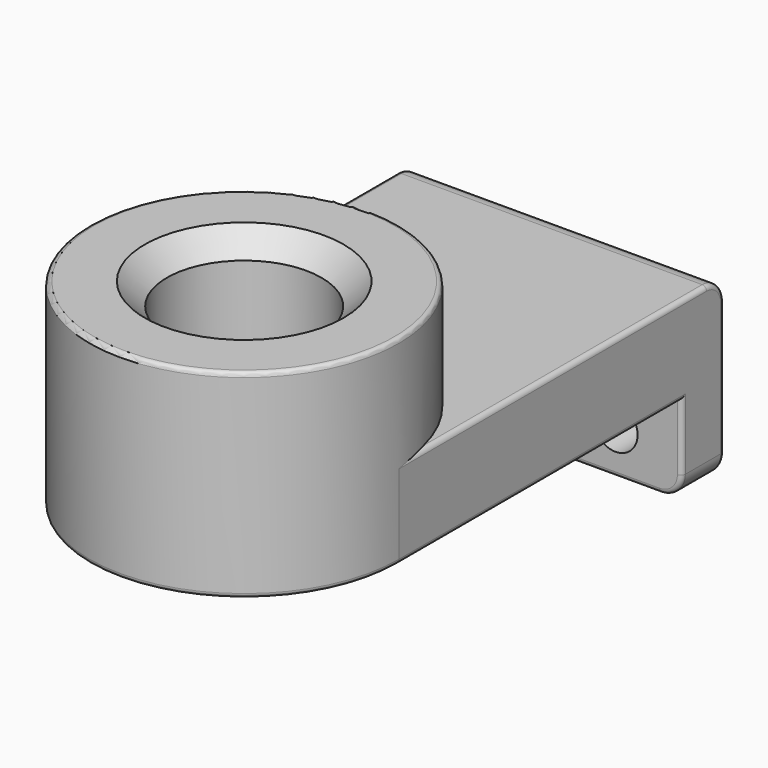
from build123d import *

# Parameters (mm, degrees)
F1_DEPTH     = 45
F2_DEPTH     = 20
F3_W         = 70
F3_H         = 20
F3_R         = 5
F4_DEPTH     = 12
F5_SIZE      = 5
F6_SIZE      = 5
F7_R         = 5
F8_T1_DEPTH  = 80
F8_T3_DEPTH  = 60
F8_T5_DEPTH  = 30
F8_T7_DEPTH  = 15
F8_T12_DEPTH = 99.5
F8_S13_R     = 35
F8_T14_DEPTH = 51
F8_T16_ANGLE = 180
F8_T20_DEPTH = 99.5
F8_S21_R     = 35
F8_T22_DEPTH = 51
F8_T24_ANGLE = 90
F8_T26_ANGLE = 90
F8_T28_ANGLE = 90
F8_T30_ANGLE = 90
F8_T32_ANGLE = 90
F8_T34_ANGLE = 90
F8_T39_DEPTH = 82.5
F8_T43_DEPTH = 17.5
F8_T50_DEPTH = 82.5
F8_T54_DEPTH = 17.5
F9_R         = 1


# Not quite as in the source:
# - a fillet or chamfer that OpenCascade refuses, or shapes differently, is made with other operations: its cross-section is extruded or revolved along the edge and cut away or added


with BuildPart() as f1:
    # F0 (on Top) → F1 (new body)
    with BuildSketch(Plane.XY):
        with BuildLine():
            Line((-23.7085466087, -49.8320348561), (-6.2085466087, -49.8320348561))
            ThreePointArc((-6.2085466087, -49.8320348561), (-41.2085466087, -14.8320348561), (-76.2085466087, -49.8320348561))
            Line((-76.2085466087, -49.8320348561), (-58.7085466087, -49.8320348561))
            ThreePointArc((-58.7085466087, -49.8320348561), (-41.2085466087, -32.3320348561), (-23.7085466087, -49.8320348561))
        make_face()
        with BuildLine():
            ThreePointArc((-76.2085466087, -49.8320348561), (-41.2085466087, -84.8320348561), (-6.2085466087, -49.8320348561))
            Line((-6.2085466087, -49.8320348561), (-23.7085466087, -49.8320348561))
            ThreePointArc((-23.7085466087, -49.8320348561), (-41.2085466087, -67.3320348561), (-58.7085466087, -49.8320348561))
            Line((-58.7085466087, -49.8320348561), (-76.2085466087, -49.8320348561))
        make_face()
    extrude(amount=F1_DEPTH)

    # F0 (on Top) → F2 (join)
    with BuildSketch(Plane.XY):
        with BuildLine():
            Line((-23.7085466087, -49.8320348561), (-6.2085466087, -49.8320348561))
            ThreePointArc((-6.2085466087, -49.8320348561), (-41.2085466087, -14.8320348561), (-76.2085466087, -49.8320348561))
            Line((-76.2085466087, -49.8320348561), (-58.7085466087, -49.8320348561))
            ThreePointArc((-58.7085466087, -49.8320348561), (-41.2085466087, -32.3320348561), (-23.7085466087, -49.8320348561))
        make_face()
        with BuildLine():
            ThreePointArc((-76.2085466087, -49.8320348561), (-41.2085466087, -84.8320348561), (-6.2085466087, -49.8320348561))
            Line((-6.2085466087, -49.8320348561), (-23.7085466087, -49.8320348561))
            ThreePointArc((-23.7085466087, -49.8320348561), (-41.2085466087, -67.3320348561), (-58.7085466087, -49.8320348561))
            Line((-58.7085466087, -49.8320348561), (-76.2085466087, -49.8320348561))
        make_face()
        with BuildLine():
            ThreePointArc((-76.2085466087, -49.8320348561), (-41.2085466087, -14.8320348561), (-6.2085466087, -49.8320348561))
            Line((-6.2085466087, -49.8320348561), (-6.2085466087, 30.1679651439))
            Line((-6.2085466087, 30.1679651439), (-76.2085466087, 30.1679651439))
            Line((-76.2085466087, 30.1679651439), (-76.2085466087, -49.8320348561))
        make_face()
    extrude(amount=F2_DEPTH)

    # F3 (on face) → F4 (join)
    with BuildSketch(Plane(origin=(0, 30.1679651439, 0), x_dir=(-1, 0, 0), z_dir=(0, 1, 0))):
        with Locations((41.2085466087, -10)):
            Rectangle(F3_W, F3_H)
        with BuildLine():
            ThreePointArc((21.2085466087, -5), (24.7440805146, -6.4644660941), (26.2085466087, -10))
            ThreePointArc((26.2085466087, -10), (17.6730127028, -13.5355339059), (21.2085466087, -5))
        make_face(mode=Mode.SUBTRACT)
        with Locations((61.2085466087, -10)):
            Circle(F3_R, mode=Mode.SUBTRACT)
        with Locations((41.2085466087, 10)):
            Rectangle(F3_W, F3_H)
    extrude(amount=F4_DEPTH)

    # F5
    f5_edges = [f1.edges().sort_by_distance(p)[0] for p in [
        (-58.708547, -49.832035, 45),
    ]]
    chamfer(f5_edges, length=F5_SIZE)

    # F6
    f6_edges = [f1.edges().sort_by_distance(p)[0] for p in [
        (-58.708547, -49.832035, 0),
    ]]
    chamfer(f6_edges, length=F6_SIZE)

    # F7
    f7_edges = [f1.edges().sort_by_distance(p)[0] for p in [
        (-76.208547, 36.167965, -20),
        (-6.208547, 36.167965, -20),
        (-41.208547, 42.167965, 20),
    ]]
    fillet(f7_edges, radius=F7_R)

    # F8: fillet of radius 1 on 9 edges, made by hand

    # F8_s2 → F8_t1 (cut)
    with BuildSketch(Plane.XZ.offset(-30.1679651439)):
        with BuildLine():
            ThreePointArc((-75.2085466087, 0), (-75.9156533899, 0.2928932188), (-76.2085466087, 1))
            Line((-76.2085466087, 1), (-76.2085466087, 0))
            Line((-76.2085466087, 0), (-75.2085466087, 0))
        make_face()
        with BuildLine():
            ThreePointArc((-6.2085466087, 1), (-6.5014398275, 0.2928932188), (-7.2085466087, 0))
            Line((-7.2085466087, 0), (-6.2085466087, 0))
            Line((-6.2085466087, 0), (-6.2085466087, 1))
        make_face()
    extrude(amount=F8_T1_DEPTH, mode=Mode.SUBTRACT)

    # F8_s4 → F8_t3 (cut)
    with BuildSketch(Plane.YZ.offset(-71.2085466087)):
        with BuildLine():
            ThreePointArc((30.1679651439, -19), (30.4608583627, -19.7071067812), (31.1679651439, -20))
            Line((31.1679651439, -20), (30.1679651439, -20))
            Line((30.1679651439, -20), (30.1679651439, -19))
        make_face()
        with BuildLine():
            ThreePointArc((42.1679651439, -19), (41.8750719251, -19.7071067812), (41.1679651439, -20))
            Line((41.1679651439, -20), (42.1679651439, -20))
            Line((42.1679651439, -20), (42.1679651439, -19))
        make_face()
    extrude(amount=F8_T3_DEPTH, mode=Mode.SUBTRACT)

    # F8_s6 → F8_t5 (cut)
    with BuildSketch(Plane.XY.offset(-15)):
        with BuildLine():
            ThreePointArc((-6.2085466087, 41.1679651439), (-6.5014398275, 41.8750719251), (-7.2085466087, 42.1679651439))
            Line((-7.2085466087, 42.1679651439), (-6.2085466087, 42.1679651439))
            Line((-6.2085466087, 42.1679651439), (-6.2085466087, 41.1679651439))
        make_face()
        with BuildLine():
            ThreePointArc((-75.2085466087, 42.1679651439), (-75.9156533899, 41.8750719251), (-76.2085466087, 41.1679651439))
            Line((-76.2085466087, 41.1679651439), (-76.2085466087, 42.1679651439))
            Line((-76.2085466087, 42.1679651439), (-75.2085466087, 42.1679651439))
        make_face()
    extrude(amount=F8_T5_DEPTH, mode=Mode.SUBTRACT)

    # F8_s8 → F8_t7 (cut)
    with BuildSketch(Plane.XY.offset(-15)):
        with BuildLine():
            ThreePointArc((-75.2085466087, 30.1679651439), (-75.9156533899, 30.4608583627), (-76.2085466087, 31.1679651439))
            Line((-76.2085466087, 31.1679651439), (-76.2085466087, 30.1679651439))
            Line((-76.2085466087, 30.1679651439), (-75.2085466087, 30.1679651439))
        make_face()
        with BuildLine():
            ThreePointArc((-6.2085466087, 31.1679651439), (-6.5014398275, 30.4608583627), (-7.2085466087, 30.1679651439))
            Line((-7.2085466087, 30.1679651439), (-6.2085466087, 30.1679651439))
            Line((-6.2085466087, 30.1679651439), (-6.2085466087, 31.1679651439))
        make_face()
    extrude(amount=F8_T7_DEPTH, mode=Mode.SUBTRACT)


with BuildPart() as f8_tool10:
    # F8_s11 → F8_t12 (new body)
    with BuildSketch(Plane.XZ.offset(62.3320348561)):
        with BuildLine():
            ThreePointArc((-75.2085466087, 20), (-75.9156533899, 19.7071067812), (-76.2085466087, 19))
            Line((-76.2085466087, 19), (-76.2085466087, 20))
            Line((-76.2085466087, 20), (-75.2085466087, 20))
        make_face()
    extrude(amount=-F8_T12_DEPTH)

    # F8_s13 → F8_t14 (cut, symmetric)
    with BuildSketch(Plane.XY.offset(19.5)):
        with Locations((-41.2085466087, -49.8320348561)):
            Circle(F8_S13_R)
    extrude(amount=F8_T14_DEPTH, both=True, mode=Mode.SUBTRACT)


with BuildPart() as f1_1:
    add(f1.part)

    # F8_t9: cut F8_tool10
    add(f8_tool10.part, mode=Mode.SUBTRACT)

    # F8_s15 → F8_t16 (revolve, cut)
    with BuildSketch(Plane.XZ.offset(49.8320348561)):
        with BuildLine():
            ThreePointArc((-76.2085466087, 1), (-75.9156533899, 0.2928932188), (-75.2085466087, 0))
            Line((-75.2085466087, 0), (-76.2085466087, 0))
            Line((-76.2085466087, 0), (-76.2085466087, 1))
        make_face()
    revolve(axis=Axis((-41.2085466087, -49.8320348561, 0), (0, 0, 1)), revolution_arc=F8_T16_ANGLE, mode=Mode.SUBTRACT)


with BuildPart() as f8_tool18:
    # F8_s19 → F8_t20 (new body)
    with BuildSketch(Plane.XZ.offset(-37.1679651439)):
        with BuildLine():
            ThreePointArc((-6.2085466087, 19), (-6.5014398275, 19.7071067812), (-7.2085466087, 20))
            Line((-7.2085466087, 20), (-6.2085466087, 20))
            Line((-6.2085466087, 20), (-6.2085466087, 19))
        make_face()
    extrude(amount=F8_T20_DEPTH)

    # F8_s21 → F8_t22 (cut, symmetric)
    with BuildSketch(Plane.XY.offset(19.5)):
        with Locations((-41.2085466087, -49.8320348561)):
            Circle(F8_S21_R)
    extrude(amount=F8_T22_DEPTH, both=True, mode=Mode.SUBTRACT)


with BuildPart() as f1_2:
    add(f1_1.part)

    # F8_t17: cut F8_tool18
    add(f8_tool18.part, mode=Mode.SUBTRACT)

    # F8_s23 → F8_t24 (revolve, cut)
    with BuildSketch(Plane.XY.offset(-15)):
        with BuildLine():
            ThreePointArc((-75.2085466087, 42.1679651439), (-75.9156533899, 41.8750719251), (-76.2085466087, 41.1679651439))
            Line((-76.2085466087, 41.1679651439), (-76.2085466087, 42.1679651439))
            Line((-76.2085466087, 42.1679651439), (-75.2085466087, 42.1679651439))
        make_face()
    revolve(axis=Axis((-71.2085466087, 42.1679651439, -15), (0, -1, 0)), revolution_arc=F8_T24_ANGLE, mode=Mode.SUBTRACT)

    # F8_s25 → F8_t26 (revolve, cut)
    with BuildSketch(Plane.XZ.offset(-37.1679651439)):
        with BuildLine():
            ThreePointArc((-75.2085466087, 20), (-75.9156533899, 19.7071067812), (-76.2085466087, 19))
            Line((-76.2085466087, 19), (-76.2085466087, 20))
            Line((-76.2085466087, 20), (-75.2085466087, 20))
        make_face()
    revolve(axis=Axis((-76.2085466087, 37.1679651439, 15), (-1, 0, 0)), revolution_arc=F8_T26_ANGLE, mode=Mode.SUBTRACT)

    # F8_s27 → F8_t28 (revolve, cut)
    with BuildSketch(Plane.XZ.offset(-37.1679651439)):
        with BuildLine():
            ThreePointArc((-6.2085466087, 19), (-6.5014398275, 19.7071067812), (-7.2085466087, 20))
            Line((-7.2085466087, 20), (-6.2085466087, 20))
            Line((-6.2085466087, 20), (-6.2085466087, 19))
        make_face()
    revolve(axis=Axis((-6.2085466087, 37.1679651439, 15), (-1, 0, 0)), revolution_arc=F8_T28_ANGLE, mode=Mode.SUBTRACT)

    # F8_s29 → F8_t30 (revolve, cut)
    with BuildSketch(Plane.XY.offset(-15)):
        with BuildLine():
            ThreePointArc((-7.2085466087, 42.1679651439), (-6.5014398275, 41.8750719251), (-6.2085466087, 41.1679651439))
            Line((-6.2085466087, 41.1679651439), (-6.2085466087, 42.1679651439))
            Line((-6.2085466087, 42.1679651439), (-7.2085466087, 42.1679651439))
        make_face()
    revolve(axis=Axis((-11.2085466087, 42.1679651439, -15), (0, 1, 0)), revolution_arc=F8_T30_ANGLE, mode=Mode.SUBTRACT)

    # F8_s31 → F8_t32 (revolve, cut)
    with BuildSketch(Plane.XY.offset(-15)):
        with BuildLine():
            ThreePointArc((-6.2085466087, 31.1679651439), (-6.5014398275, 30.4608583627), (-7.2085466087, 30.1679651439))
            Line((-7.2085466087, 30.1679651439), (-6.2085466087, 30.1679651439))
            Line((-6.2085466087, 30.1679651439), (-6.2085466087, 31.1679651439))
        make_face()
    revolve(axis=Axis((-11.2085466087, 30.1679651439, -15), (0, 1, 0)), revolution_arc=F8_T32_ANGLE, mode=Mode.SUBTRACT)

    # F8_s33 → F8_t34 (revolve, cut)
    with BuildSketch(Plane.XY.offset(-15)):
        with BuildLine():
            ThreePointArc((-75.2085466087, 30.1679651439), (-75.9156533899, 30.4608583627), (-76.2085466087, 31.1679651439))
            Line((-76.2085466087, 31.1679651439), (-76.2085466087, 30.1679651439))
            Line((-76.2085466087, 30.1679651439), (-75.2085466087, 30.1679651439))
        make_face()
    revolve(axis=Axis((-71.2085466087, 30.1679651439, -15), (0, -1, 0)), revolution_arc=F8_T34_ANGLE, mode=Mode.SUBTRACT)


with BuildPart() as f8_tool37:
    # F8_s38 → F8_t39 (new body)
    with BuildSketch(Plane.XZ.offset(-32.6679651439)):
        with BuildLine():
            ThreePointArc((-75.2085466087, 0), (-75.9156533899, 0.2928932188), (-76.2085466087, 1))
            Line((-76.2085466087, 1), (-76.2085466087, 0))
            Line((-76.2085466087, 0), (-75.2085466087, 0))
        make_face()
    extrude(amount=F8_T39_DEPTH)

    split(bisect_by=Plane.XZ.offset(-30.1679651439), keep=Keep.BOTTOM)


with BuildPart() as f8_tool41:
    # F8_s42 → F8_t43 (new body)
    with BuildSketch(Plane.XY.offset(-15)):
        with BuildLine():
            ThreePointArc((-75.2085466087, 30.1679651439), (-75.9156533899, 30.4608583627), (-76.2085466087, 31.1679651439))
            Line((-76.2085466087, 31.1679651439), (-76.2085466087, 30.1679651439))
            Line((-76.2085466087, 30.1679651439), (-75.2085466087, 30.1679651439))
        make_face()
    extrude(amount=F8_T43_DEPTH)

    split(bisect_by=Plane.XY, keep=Keep.TOP)


with BuildPart() as f8_tool37_1:
    add(f8_tool37.part)

    # F8_t45: intersect F8_tool41
    add(f8_tool41.part, mode=Mode.INTERSECT)


with BuildPart() as f1_3:
    add(f1_2.part)

    # F8_t35: cut F8_tool37
    add(f8_tool37_1.part, mode=Mode.SUBTRACT)


with BuildPart() as f8_tool48:
    # F8_s49 → F8_t50 (new body)
    with BuildSketch(Plane.XZ.offset(49.8320348561)):
        with BuildLine():
            ThreePointArc((-6.2085466087, 1), (-6.5014398275, 0.2928932188), (-7.2085466087, 0))
            Line((-7.2085466087, 0), (-6.2085466087, 0))
            Line((-6.2085466087, 0), (-6.2085466087, 1))
        make_face()
    extrude(amount=-F8_T50_DEPTH)

    split(bisect_by=Plane.XZ.offset(-30.1679651439), keep=Keep.BOTTOM)


with BuildPart() as f8_tool52:
    # F8_s53 → F8_t54 (new body)
    with BuildSketch(Plane.XY.offset(2.5)):
        with BuildLine():
            ThreePointArc((-6.2085466087, 31.1679651439), (-6.5014398275, 30.4608583627), (-7.2085466087, 30.1679651439))
            Line((-7.2085466087, 30.1679651439), (-6.2085466087, 30.1679651439))
            Line((-6.2085466087, 30.1679651439), (-6.2085466087, 31.1679651439))
        make_face()
    extrude(amount=-F8_T54_DEPTH)

    split(bisect_by=Plane.XY, keep=Keep.TOP)


with BuildPart() as f8_tool48_1:
    add(f8_tool48.part)

    # F8_t56: intersect F8_tool52
    add(f8_tool52.part, mode=Mode.INTERSECT)


with BuildPart() as f1_4:
    add(f1_3.part)

    # F8_t46: cut F8_tool48
    add(f8_tool48_1.part, mode=Mode.SUBTRACT)

    # F9
    f9_edges = [f1_4.edges().sort_by_distance(p)[0] for p in [
        (-6.208547, -49.832035, 45),
    ]]
    fillet(f9_edges, radius=F9_R)


solid = f1_4.part
